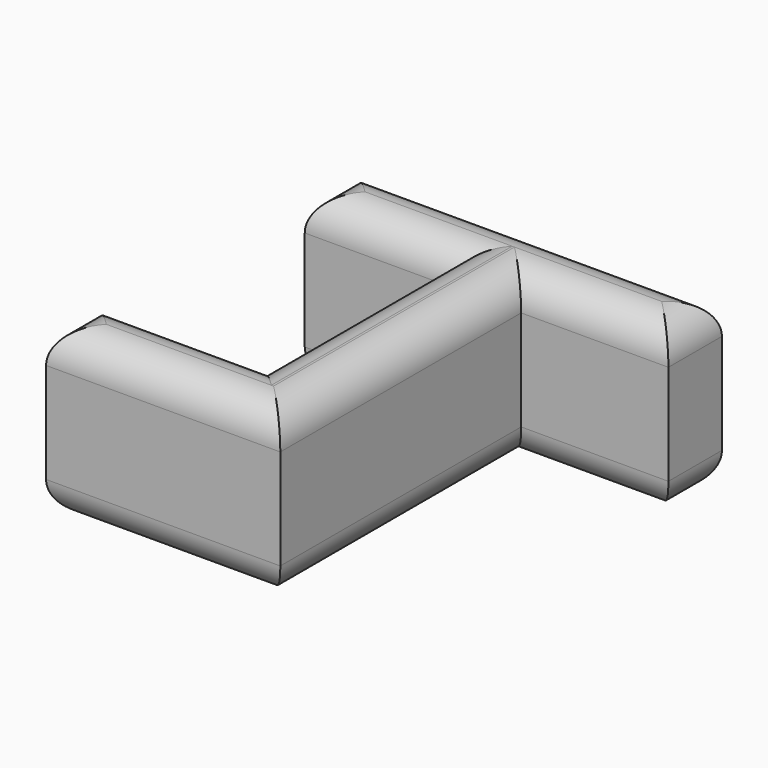
from build123d import *

# Parameters (mm, degrees)
F1_DEPTH = 25
F2_R     = 4.99999


# Not quite as in the source:
# - a fillet or chamfer is up to 0.001 mm smaller than in the source, because OpenCascade refuses the exact size


with BuildPart() as f1:
    # F0 (on Top) → F1 (new body)
    with BuildSketch(Plane.XY):
        Polygon((-35, 0), (0, 0), (0, 45), (22, 45), (22, 55), (-32.3444679379, 55), (-32.3444679379, 45), (-10.3444679379, 45), (-10.3444679379, 10), (-35, 10), align=None)
    extrude(amount=F1_DEPTH)

    # F2 (radius 5 in the source; OpenCascade refuses exactly that, so slightly less here)
    f2_edges = [f1.edges().sort_by_distance(p)[0] for p in [
        (-5.172234, 55, 0),
        (-32.344468, 50, 0),
        (-10.344468, 27.5, 0),
        (-21.344468, 45, 0),
        (11, 45, 0),
        (22, 50, 0),
        (0, 22.5, 0),
        (-17.5, 0, 0),
        (-22.672234, 10, 0),
        (-35, 5, 0),
        (-5.172234, 55, 25),
        (11, 45, 25),
        (-21.344468, 45, 25),
        (-32.344468, 50, 25),
        (22, 50, 25),
        (-10.344468, 27.5, 25),
        (-22.672234, 10, 25),
        (-35, 5, 25),
        (-17.5, 0, 25),
        (0, 22.5, 25),
    ]]
    fillet(f2_edges, radius=F2_R)


solid = f1.part
